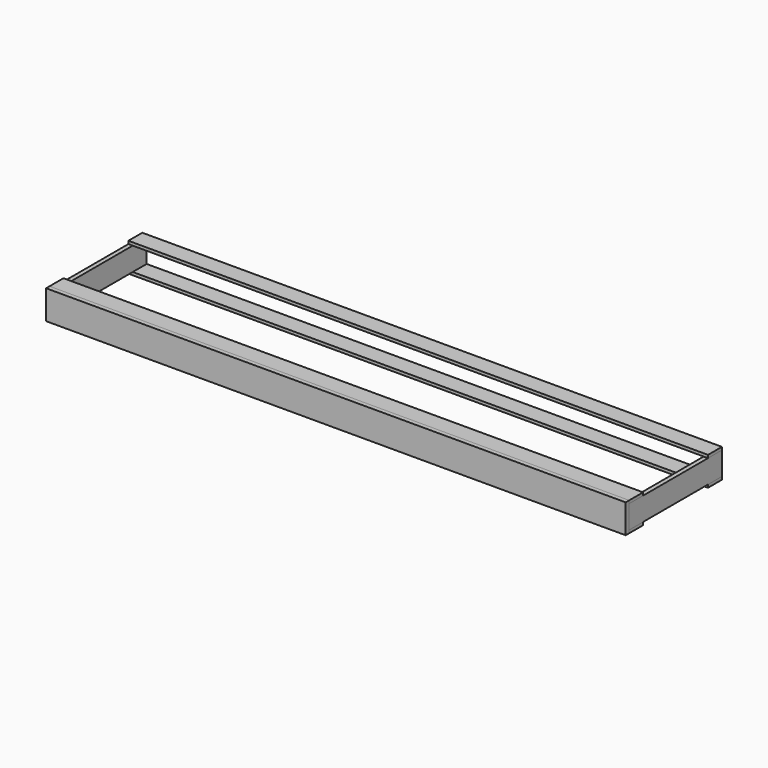
from build123d import *

# Parameters (mm, degrees)
F1_W      = 508
F1_H      = 101.6
F2_DEPTH  = 19.05
F3_W      = 76.2
F3_H      = 12.7
F5_DEPTH  = 2540
F8_W      = 508
F8_H      = 101.6
F9_DEPTH  = 19.05
F10_W     = 2539.9999999998
F10_H     = 127
F11_DEPTH = 19.05


# Not quite as in the source:
# - a variable given as a bare number and used for a length is read in inches; the dataset says mm whatever the document's units were


with BuildPart() as f2:
    # F1 (on Right) → F2 (new body)
    with BuildSketch(Plane.YZ):
        with Locations((254, 63.5)):
            Rectangle(F1_W, F1_H)
    extrude(amount=-F2_DEPTH)


with BuildPart() as f5:
    # F3 (on Right) → F5 (new body, through all)
    with BuildSketch(Plane.YZ):
        with Locations((38.1, 120.65)):
            Rectangle(F3_W, F3_H)
    extrude(amount=-F5_DEPTH)


with BuildPart() as f5b:
    # F3 (on Right) → F5, piece 2 (new body, through all)
    with BuildSketch(Plane.YZ):
        with Locations((38.1, 6.35)):
            Rectangle(F3_W, F3_H)
    extrude(amount=-F5_DEPTH)


with BuildPart() as f5c:
    # F3 (on Right) → F5, piece 3 (new body, through all)
    with BuildSketch(Plane.YZ):
        with Locations((469.9, 6.35)):
            Rectangle(F3_W, F3_H)
    extrude(amount=-F5_DEPTH)


with BuildPart() as f5d:
    # F3 (on Right) → F5, piece 4 (new body, through all)
    with BuildSketch(Plane.YZ):
        with Locations((469.9, 120.65)):
            Rectangle(F3_W, F3_H)
    extrude(amount=-F5_DEPTH)


with BuildPart() as f6_1:
    # F6: copy of F2
    add(f2.part.moved(Location((-891.54, 0, 0))))


with BuildPart() as f9:
    # F8 (on offset) → F9 (new body)
    with BuildSketch(Plane.YZ.offset(-2540)):
        with Locations((254, 63.5)):
            Rectangle(F8_W, F8_H)
    extrude(amount=F9_DEPTH)


with BuildPart() as f11:
    # F10 (on face) → F11 (new body)
    with BuildSketch(Plane.XZ):
        with Locations((-1270.0000000002, 63.5)):
            Rectangle(F10_W, F10_H)
    extrude(amount=F11_DEPTH)


solid = Compound([f2.part, f5.part, f5b.part, f5c.part, f5d.part, f9.part, f11.part])
